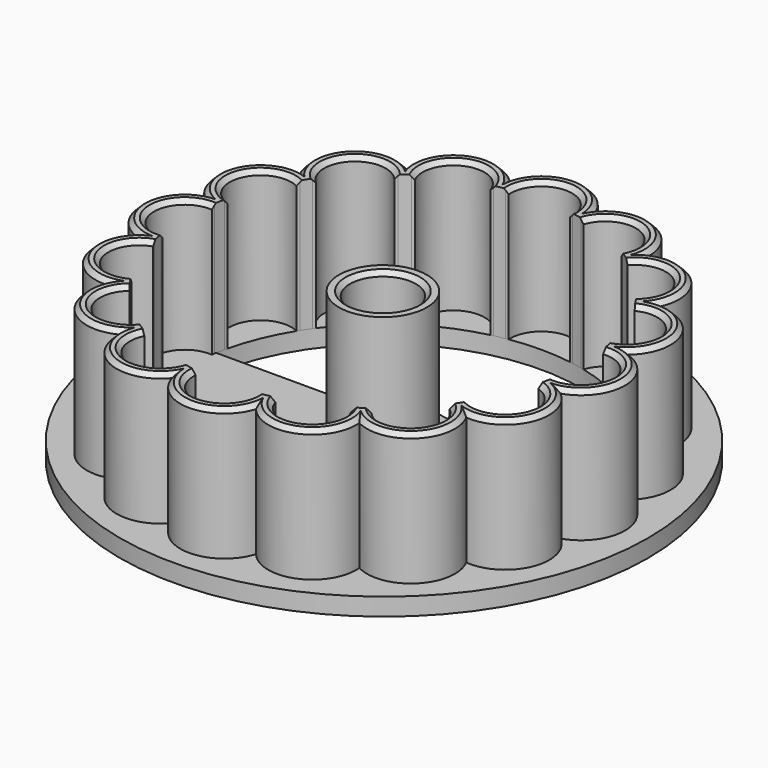
from build123d import *

# Parameters (mm, degrees)
F0_R     = 30
F0_R_2   = 3.75
F1_DEPTH = 2
F2_R     = 5
F2_R_2   = 3.75
F3_DEPTH = 15
F4_SIZE  = 0.5


with BuildPart() as f1:
    # F0 (on Top) → F1 (new body)
    with BuildSketch(Plane.XY):
        with Locations((0, 0.1543397957)):
            Circle(F0_R)
        with BuildLine():
            ThreePointArc((22.1415898255, 4), (22.4102183286, 2.0080125655), (22.5, 0))
            ThreePointArc((22.5, 0), (22.4102183286, -2.0080125655), (22.1415898255, -4))
            ThreePointArc((22.1415898255, -4), (0, -22.5), (-22.1415898255, -4))
            ThreePointArc((-22.1415898255, -4), (-22.5, 0), (-22.1415898255, 4))
            ThreePointArc((-22.1415898255, 4), (0, 22.5), (22.1415898255, 4))
        make_face(mode=Mode.SUBTRACT)
        with BuildLine():
            ThreePointArc((22.1415898255, -4), (22.4102183286, -2.0080125655), (22.5, 0))
            ThreePointArc((22.5, 0), (22.4102183286, 2.0080125655), (22.1415898255, 4))
            Line((22.1415898255, 4), (5.8490082572, 4))
            ThreePointArc((5.8490082572, 4), (0, 7.1543397957), (-5.8490082572, 4))
            Line((-5.8490082572, 4), (-22.1415898255, 4))
            ThreePointArc((-22.1415898255, 4), (-22.5, 0), (-22.1415898255, -4))
            Line((-22.1415898255, -4), (-5.6339560579, -4))
            ThreePointArc((-5.6339560579, -4), (0, -6.8456602043), (5.6339560579, -4))
            Line((5.6339560579, -4), (22.1415898255, -4))
        make_face()
        Circle(F0_R_2, mode=Mode.SUBTRACT)
    extrude(amount=F1_DEPTH)

    # F2 (on face) → F3 (join)
    with BuildSketch(Plane.XY.offset(2)):
        with BuildLine():
            ThreePointArc((3.8069810153, -22.1755923382), (3.6482825778, -22.2022529089), (3.4893975213, -22.2277777778))
            ThreePointArc((3.4893975213, -22.2277777778), (0, -26), (-3.4893975213, -22.2277777778))
            ThreePointArc((-3.4893975213, -22.2277777778), (-3.6482825778, -22.2022529089), (-3.8069810153, -22.1755923382))
            ThreePointArc((-3.8069810153, -22.1755923382), (-4.1952253001, -23.1338685771), (-4.7722662453, -23.991802562))
            ThreePointArc((-4.7722662453, -23.991802562), (0, -27.5), (4.7722662453, -23.991802562))
            ThreePointArc((4.7722662453, -23.991802562), (4.1952253001, -23.1338685771), (3.8069810153, -22.1755923382))
        make_face()
        with BuildLine():
            ThreePointArc((4.96903995, -21.9444444444), (4.3895322454, -22.0676688091), (3.8069810153, -22.1755923382))
            ThreePointArc((3.8069810153, -22.1755923382), (4.1952253001, -23.1338685771), (4.7722662453, -23.991802562))
            ThreePointArc((4.7722662453, -23.991802562), (4.9770654419, -22.9783509036), (4.96903995, -21.9444444444))
        make_face()
        with BuildLine():
            ThreePointArc((5.2824193431, -21.8711235624), (5.125860747, -21.9083443373), (4.96903995, -21.9444444444))
            ThreePointArc((4.96903995, -21.9444444444), (4.9770654419, -22.9783509036), (4.7722662453, -23.991802562))
            ThreePointArc((4.7722662453, -23.991802562), (10.52379439, -25.4066871441), (13.5902644608, -20.3392681081))
            ThreePointArc((13.5902644608, -20.3392681081), (12.72883102, -19.7674644688), (12.0034236314, -19.0307073207))
            ThreePointArc((12.0034236314, -19.0307073207), (11.8670079519, -19.1160697391), (11.7299852446, -19.2004543218))
            ThreePointArc((11.7299852446, -19.2004543218), (9.9497692415, -24.0208678453), (5.2824193431, -21.8711235624))
        make_face()
        with BuildLine():
            ThreePointArc((-4.7722662453, -23.991802562), (-4.1952253001, -23.1338685771), (-3.8069810153, -22.1755923382))
            ThreePointArc((-3.8069810153, -22.1755923382), (-4.3895322454, -22.0676688091), (-4.96903995, -21.9444444444))
            ThreePointArc((-4.96903995, -21.9444444444), (-4.9770654419, -22.9783509036), (-4.7722662453, -23.991802562))
        make_face()
        with BuildLine():
            ThreePointArc((-13.5902644608, -20.3392681081), (-10.52379439, -25.4066871441), (-4.7722662453, -23.991802562))
            ThreePointArc((-4.7722662453, -23.991802562), (-4.9770654419, -22.9783509036), (-4.96903995, -21.9444444444))
            ThreePointArc((-4.96903995, -21.9444444444), (-5.125860747, -21.9083443373), (-5.2824193431, -21.8711235624))
            ThreePointArc((-5.2824193431, -21.8711235624), (-9.9497692415, -24.0208678453), (-11.7299852446, -19.2004543218))
            ThreePointArc((-11.7299852446, -19.2004543218), (-11.8670079519, -19.1160697391), (-12.0034236314, -19.0307073207))
            ThreePointArc((-12.0034236314, -19.0307073207), (-12.72883102, -19.7674644688), (-13.5902644608, -20.3392681081))
        make_face()
        with BuildLine():
            ThreePointArc((12.0034236314, -19.0307073207), (12.72883102, -19.7674644688), (13.5902644608, -20.3392681081))
            ThreePointArc((13.5902644608, -20.3392681081), (13.3916430876, -19.3245876043), (12.9885696274, -18.3724538109))
            ThreePointArc((12.9885696274, -18.3724538109), (12.5003302429, -18.7080662768), (12.0034236314, -19.0307073207))
        make_face()
        with BuildLine():
            ThreePointArc((12.9885696274, -18.3724538109), (13.3916430876, -19.3245876043), (13.5902644608, -20.3392681081))
            ThreePointArc((13.5902644608, -20.3392681081), (19.4454364826, -19.4454364826), (20.3392681081, -13.5902644608))
            ThreePointArc((20.3392681081, -13.5902644608), (19.3245876043, -13.3916430876), (18.3724538109, -12.9885696274))
            ThreePointArc((18.3724538109, -12.9885696274), (18.27908894, -13.1196382391), (18.1847890469, -13.2500357478))
            ThreePointArc((18.1847890469, -13.2500357478), (18.3847763109, -18.3847763109), (13.2500357478, -18.1847890469))
            ThreePointArc((13.2500357478, -18.1847890469), (13.1196382391, -18.27908894), (12.9885696274, -18.3724538109))
        make_face()
        with BuildLine():
            ThreePointArc((-12.9885696274, -18.3724538109), (-13.3916430876, -19.3245876043), (-13.5902644608, -20.3392681081))
            ThreePointArc((-13.5902644608, -20.3392681081), (-12.72883102, -19.7674644688), (-12.0034236314, -19.0307073207))
            ThreePointArc((-12.0034236314, -19.0307073207), (-12.5003302429, -18.7080662768), (-12.9885696274, -18.3724538109))
        make_face()
        with BuildLine():
            ThreePointArc((-20.3392681081, -13.5902644608), (-19.4454364826, -19.4454364826), (-13.5902644608, -20.3392681081))
            ThreePointArc((-13.5902644608, -20.3392681081), (-13.3916430876, -19.3245876043), (-12.9885696274, -18.3724538109))
            ThreePointArc((-12.9885696274, -18.3724538109), (-13.1196382391, -18.27908894), (-13.2500357478, -18.1847890469))
            ThreePointArc((-13.2500357478, -18.1847890469), (-18.3847763109, -18.3847763109), (-18.1847890469, -13.2500357478))
            ThreePointArc((-18.1847890469, -13.2500357478), (-18.27908894, -13.1196382391), (-18.3724538109, -12.9885696274))
            ThreePointArc((-18.3724538109, -12.9885696274), (-19.3245876043, -13.3916430876), (-20.3392681081, -13.5902644608))
        make_face()
        with BuildLine():
            ThreePointArc((18.3724538109, -12.9885696274), (19.3245876043, -13.3916430876), (20.3392681081, -13.5902644608))
            ThreePointArc((20.3392681081, -13.5902644608), (19.7674644688, -12.72883102), (19.0307073207, -12.0034236314))
            ThreePointArc((19.0307073207, -12.0034236314), (18.7080662768, -12.5003302429), (18.3724538109, -12.9885696274))
        make_face()
        with BuildLine():
            ThreePointArc((19.0307073207, -12.0034236314), (19.7674644688, -12.72883102), (20.3392681081, -13.5902644608))
            ThreePointArc((20.3392681081, -13.5902644608), (25.4066871441, -10.52379439), (23.991802562, -4.7722662453))
            ThreePointArc((23.991802562, -4.7722662453), (22.9783509036, -4.9770654419), (21.9444444444, -4.96903995))
            ThreePointArc((21.9444444444, -4.96903995), (21.9083443373, -5.125860747), (21.8711235624, -5.2824193431))
            ThreePointArc((21.8711235624, -5.2824193431), (24.0208678453, -9.9497692415), (19.2004543218, -11.7299852446))
            ThreePointArc((19.2004543218, -11.7299852446), (19.1160697391, -11.8670079519), (19.0307073207, -12.0034236314))
        make_face()
        with BuildLine():
            ThreePointArc((-19.0307073207, -12.0034236314), (-19.7674644688, -12.72883102), (-20.3392681081, -13.5902644608))
            ThreePointArc((-20.3392681081, -13.5902644608), (-19.3245876043, -13.3916430876), (-18.3724538109, -12.9885696274))
            ThreePointArc((-18.3724538109, -12.9885696274), (-18.7080662768, -12.5003302429), (-19.0307073207, -12.0034236314))
        make_face()
        with BuildLine():
            ThreePointArc((-23.991802562, -4.7722662453), (-25.4066871441, -10.52379439), (-20.3392681081, -13.5902644608))
            ThreePointArc((-20.3392681081, -13.5902644608), (-19.7674644688, -12.72883102), (-19.0307073207, -12.0034236314))
            ThreePointArc((-19.0307073207, -12.0034236314), (-19.1160697391, -11.8670079519), (-19.2004543218, -11.7299852446))
            ThreePointArc((-19.2004543218, -11.7299852446), (-24.0208678453, -9.9497692415), (-21.8711235624, -5.2824193431))
            ThreePointArc((-21.8711235624, -5.2824193431), (-21.9083443373, -5.125860747), (-21.9444444444, -4.96903995))
            ThreePointArc((-21.9444444444, -4.96903995), (-22.9783509036, -4.9770654419), (-23.991802562, -4.7722662453))
        make_face()
        with BuildLine():
            ThreePointArc((21.9444444444, -4.96903995), (22.9783509036, -4.9770654419), (23.991802562, -4.7722662453))
            ThreePointArc((23.991802562, -4.7722662453), (23.1338685771, -4.1952253001), (22.1755923382, -3.8069810153))
            ThreePointArc((22.1755923382, -3.8069810153), (22.0676688091, -4.3895322454), (21.9444444444, -4.96903995))
        make_face()
        with BuildLine():
            ThreePointArc((22.1755923382, -3.8069810153), (23.1338685771, -4.1952253001), (23.991802562, -4.7722662453))
            ThreePointArc((23.991802562, -4.7722662453), (27.5, 0), (23.991802562, 4.7722662453))
            ThreePointArc((23.991802562, 4.7722662453), (23.1338685771, 4.1952253001), (22.1755923382, 3.8069810153))
            ThreePointArc((22.1755923382, 3.8069810153), (22.2022529089, 3.6482825778), (22.2277777778, 3.4893975213))
            ThreePointArc((22.2277777778, 3.4893975213), (26, 0), (22.2277777778, -3.4893975213))
            ThreePointArc((22.2277777778, -3.4893975213), (22.2022529089, -3.6482825778), (22.1755923382, -3.8069810153))
        make_face()
        with BuildLine():
            ThreePointArc((-22.1755923382, -3.8069810153), (-23.1338685771, -4.1952253001), (-23.991802562, -4.7722662453))
            ThreePointArc((-23.991802562, -4.7722662453), (-22.9783509036, -4.9770654419), (-21.9444444444, -4.96903995))
            ThreePointArc((-21.9444444444, -4.96903995), (-22.0676688091, -4.3895322454), (-22.1755923382, -3.8069810153))
        make_face()
        with BuildLine():
            ThreePointArc((-23.991802562, 4.7722662453), (-27.5, 0), (-23.991802562, -4.7722662453))
            ThreePointArc((-23.991802562, -4.7722662453), (-23.1338685771, -4.1952253001), (-22.1755923382, -3.8069810153))
            ThreePointArc((-22.1755923382, -3.8069810153), (-22.2022529089, -3.6482825778), (-22.2277777778, -3.4893975213))
            ThreePointArc((-22.2277777778, -3.4893975213), (-26, 0), (-22.2277777778, 3.4893975213))
            ThreePointArc((-22.2277777778, 3.4893975213), (-22.2022529089, 3.6482825778), (-22.1755923382, 3.8069810153))
            ThreePointArc((-22.1755923382, 3.8069810153), (-23.1338685771, 4.1952253001), (-23.991802562, 4.7722662453))
        make_face()
        with BuildLine():
            ThreePointArc((22.1755923382, 3.8069810153), (23.1338685771, 4.1952253001), (23.991802562, 4.7722662453))
            ThreePointArc((23.991802562, 4.7722662453), (22.9783509036, 4.9770654419), (21.9444444444, 4.96903995))
            ThreePointArc((21.9444444444, 4.96903995), (22.0676688091, 4.3895322454), (22.1755923382, 3.8069810153))
        make_face()
        with BuildLine():
            ThreePointArc((21.9444444444, 4.96903995), (22.9783509036, 4.9770654419), (23.991802562, 4.7722662453))
            ThreePointArc((23.991802562, 4.7722662453), (25.4066871441, 10.52379439), (20.3392681081, 13.5902644608))
            ThreePointArc((20.3392681081, 13.5902644608), (19.7674644688, 12.72883102), (19.0307073207, 12.0034236314))
            ThreePointArc((19.0307073207, 12.0034236314), (19.1160697391, 11.8670079519), (19.2004543218, 11.7299852446))
            ThreePointArc((19.2004543218, 11.7299852446), (24.0208678453, 9.9497692415), (21.8711235624, 5.2824193431))
            ThreePointArc((21.8711235624, 5.2824193431), (21.9083443373, 5.125860747), (21.9444444444, 4.96903995))
        make_face()
        with BuildLine():
            ThreePointArc((-21.9444444444, 4.96903995), (-22.9783509036, 4.9770654419), (-23.991802562, 4.7722662453))
            ThreePointArc((-23.991802562, 4.7722662453), (-23.1338685771, 4.1952253001), (-22.1755923382, 3.8069810153))
            ThreePointArc((-22.1755923382, 3.8069810153), (-22.0676688091, 4.3895322454), (-21.9444444444, 4.96903995))
        make_face()
        with BuildLine():
            ThreePointArc((-20.3392681081, 13.5902644608), (-25.4066871441, 10.52379439), (-23.991802562, 4.7722662453))
            ThreePointArc((-23.991802562, 4.7722662453), (-22.9783509036, 4.9770654419), (-21.9444444444, 4.96903995))
            ThreePointArc((-21.9444444444, 4.96903995), (-21.9083443373, 5.125860747), (-21.8711235624, 5.2824193431))
            ThreePointArc((-21.8711235624, 5.2824193431), (-24.0208678453, 9.9497692415), (-19.2004543218, 11.7299852446))
            ThreePointArc((-19.2004543218, 11.7299852446), (-19.1160697391, 11.8670079519), (-19.0307073207, 12.0034236314))
            ThreePointArc((-19.0307073207, 12.0034236314), (-19.7674644688, 12.72883102), (-20.3392681081, 13.5902644608))
        make_face()
        with BuildLine():
            ThreePointArc((19.0307073207, 12.0034236314), (19.7674644688, 12.72883102), (20.3392681081, 13.5902644608))
            ThreePointArc((20.3392681081, 13.5902644608), (19.3245876043, 13.3916430876), (18.3724538109, 12.9885696274))
            ThreePointArc((18.3724538109, 12.9885696274), (18.7080662768, 12.5003302429), (19.0307073207, 12.0034236314))
        make_face()
        with BuildLine():
            ThreePointArc((18.3724538109, 12.9885696274), (19.3245876043, 13.3916430876), (20.3392681081, 13.5902644608))
            ThreePointArc((20.3392681081, 13.5902644608), (19.4454364826, 19.4454364826), (13.5902644608, 20.3392681081))
            ThreePointArc((13.5902644608, 20.3392681081), (13.3916430876, 19.3245876043), (12.9885696274, 18.3724538109))
            ThreePointArc((12.9885696274, 18.3724538109), (13.1196382391, 18.27908894), (13.2500357478, 18.1847890469))
            ThreePointArc((13.2500357478, 18.1847890469), (18.3847763109, 18.3847763109), (18.1847890469, 13.2500357478))
            ThreePointArc((18.1847890469, 13.2500357478), (18.27908894, 13.1196382391), (18.3724538109, 12.9885696274))
        make_face()
        with BuildLine():
            ThreePointArc((-18.3724538109, 12.9885696274), (-19.3245876043, 13.3916430876), (-20.3392681081, 13.5902644608))
            ThreePointArc((-20.3392681081, 13.5902644608), (-19.7674644688, 12.72883102), (-19.0307073207, 12.0034236314))
            ThreePointArc((-19.0307073207, 12.0034236314), (-18.7080662768, 12.5003302429), (-18.3724538109, 12.9885696274))
        make_face()
        with BuildLine():
            ThreePointArc((-13.5902644608, 20.3392681081), (-19.4454364826, 19.4454364826), (-20.3392681081, 13.5902644608))
            ThreePointArc((-20.3392681081, 13.5902644608), (-19.3245876043, 13.3916430876), (-18.3724538109, 12.9885696274))
            ThreePointArc((-18.3724538109, 12.9885696274), (-18.27908894, 13.1196382391), (-18.1847890469, 13.2500357478))
            ThreePointArc((-18.1847890469, 13.2500357478), (-18.3847763109, 18.3847763109), (-13.2500357478, 18.1847890469))
            ThreePointArc((-13.2500357478, 18.1847890469), (-13.1196382391, 18.27908894), (-12.9885696274, 18.3724538109))
            ThreePointArc((-12.9885696274, 18.3724538109), (-13.3916430876, 19.3245876043), (-13.5902644608, 20.3392681081))
        make_face()
        with BuildLine():
            ThreePointArc((12.9885696274, 18.3724538109), (13.3916430876, 19.3245876043), (13.5902644608, 20.3392681081))
            ThreePointArc((13.5902644608, 20.3392681081), (12.72883102, 19.7674644688), (12.0034236314, 19.0307073207))
            ThreePointArc((12.0034236314, 19.0307073207), (12.5003302429, 18.7080662768), (12.9885696274, 18.3724538109))
        make_face()
        with BuildLine():
            ThreePointArc((12.0034236314, 19.0307073207), (12.72883102, 19.7674644688), (13.5902644608, 20.3392681081))
            ThreePointArc((13.5902644608, 20.3392681081), (10.52379439, 25.4066871441), (4.7722662453, 23.991802562))
            ThreePointArc((4.7722662453, 23.991802562), (4.9770654419, 22.9783509036), (4.96903995, 21.9444444444))
            ThreePointArc((4.96903995, 21.9444444444), (5.125860747, 21.9083443373), (5.2824193431, 21.8711235624))
            ThreePointArc((5.2824193431, 21.8711235624), (9.9497692415, 24.0208678453), (11.7299852446, 19.2004543218))
            ThreePointArc((11.7299852446, 19.2004543218), (11.8670079519, 19.1160697391), (12.0034236314, 19.0307073207))
        make_face()
        with BuildLine():
            ThreePointArc((-12.0034236314, 19.0307073207), (-12.72883102, 19.7674644688), (-13.5902644608, 20.3392681081))
            ThreePointArc((-13.5902644608, 20.3392681081), (-13.3916430876, 19.3245876043), (-12.9885696274, 18.3724538109))
            ThreePointArc((-12.9885696274, 18.3724538109), (-12.5003302429, 18.7080662768), (-12.0034236314, 19.0307073207))
        make_face()
        with BuildLine():
            ThreePointArc((-4.7722662453, 23.991802562), (-10.52379439, 25.4066871441), (-13.5902644608, 20.3392681081))
            ThreePointArc((-13.5902644608, 20.3392681081), (-12.72883102, 19.7674644688), (-12.0034236314, 19.0307073207))
            ThreePointArc((-12.0034236314, 19.0307073207), (-11.8670079519, 19.1160697391), (-11.7299852446, 19.2004543218))
            ThreePointArc((-11.7299852446, 19.2004543218), (-9.9497692415, 24.0208678453), (-5.2824193431, 21.8711235624))
            ThreePointArc((-5.2824193431, 21.8711235624), (-5.125860747, 21.9083443373), (-4.96903995, 21.9444444444))
            ThreePointArc((-4.96903995, 21.9444444444), (-4.9770654419, 22.9783509036), (-4.7722662453, 23.991802562))
        make_face()
        with BuildLine():
            ThreePointArc((4.96903995, 21.9444444444), (4.9770654419, 22.9783509036), (4.7722662453, 23.991802562))
            ThreePointArc((4.7722662453, 23.991802562), (4.1952253001, 23.1338685771), (3.8069810153, 22.1755923382))
            ThreePointArc((3.8069810153, 22.1755923382), (4.3895322454, 22.0676688091), (4.96903995, 21.9444444444))
        make_face()
        with BuildLine():
            ThreePointArc((3.8069810153, 22.1755923382), (4.1952253001, 23.1338685771), (4.7722662453, 23.991802562))
            ThreePointArc((4.7722662453, 23.991802562), (0, 27.5), (-4.7722662453, 23.991802562))
            ThreePointArc((-4.7722662453, 23.991802562), (-4.1952253001, 23.1338685771), (-3.8069810153, 22.1755923382))
            ThreePointArc((-3.8069810153, 22.1755923382), (-3.6482825778, 22.2022529089), (-3.4893975213, 22.2277777778))
            ThreePointArc((-3.4893975213, 22.2277777778), (0, 26), (3.4893975213, 22.2277777778))
            ThreePointArc((3.4893975213, 22.2277777778), (3.6482825778, 22.2022529089), (3.8069810153, 22.1755923382))
        make_face()
        with BuildLine():
            ThreePointArc((-3.8069810153, 22.1755923382), (-4.1952253001, 23.1338685771), (-4.7722662453, 23.991802562))
            ThreePointArc((-4.7722662453, 23.991802562), (-4.9770654419, 22.9783509036), (-4.96903995, 21.9444444444))
            ThreePointArc((-4.96903995, 21.9444444444), (-4.3895322454, 22.0676688091), (-3.8069810153, 22.1755923382))
        make_face()
        Circle(F2_R)
        Circle(F2_R_2, mode=Mode.SUBTRACT)
    extrude(amount=F3_DEPTH)

    # F4
    f4_edges = [f1.edges().sort_by_distance(p)[0] for p in [
        (-10.523794, 25.406687, 17),
        (0, 27.5, 17),
        (10.523794, 25.406687, 17),
        (19.445436, 19.445436, 17),
        (25.406687, 10.523794, 17),
        (27.5, 0, 17),
        (25.406687, -10.523794, 17),
        (19.445436, -19.445436, 17),
        (10.523794, -25.406687, 17),
        (0, -27.5, 17),
        (-10.523794, -25.406687, 17),
        (-19.445436, -19.445436, 17),
        (-25.406687, -10.523794, 17),
        (-27.5, 0, 17),
        (-25.406687, 10.523794, 17),
        (-19.445436, 19.445436, 17),
        (-18.384776, 18.384776, 17),
        (-9.949769, 24.020868, 17),
        (0, 26, 17),
        (9.949769, 24.020868, 17),
        (18.384776, 18.384776, 17),
        (24.020868, 9.949769, 17),
        (26, 0, 17),
        (24.020868, -9.949769, 17),
        (18.384776, -18.384776, 17),
        (9.949769, -24.020868, 17),
        (0, -26, 17),
        (-9.949769, -24.020868, 17),
        (-18.384776, -18.384776, 17),
        (-24.020868, -9.949769, 17),
        (-26, 0, 17),
        (-24.020868, 9.949769, 17),
        (-3.75, 0, 17),
    ]]
    chamfer(f4_edges, length=F4_SIZE)


solid = f1.part
